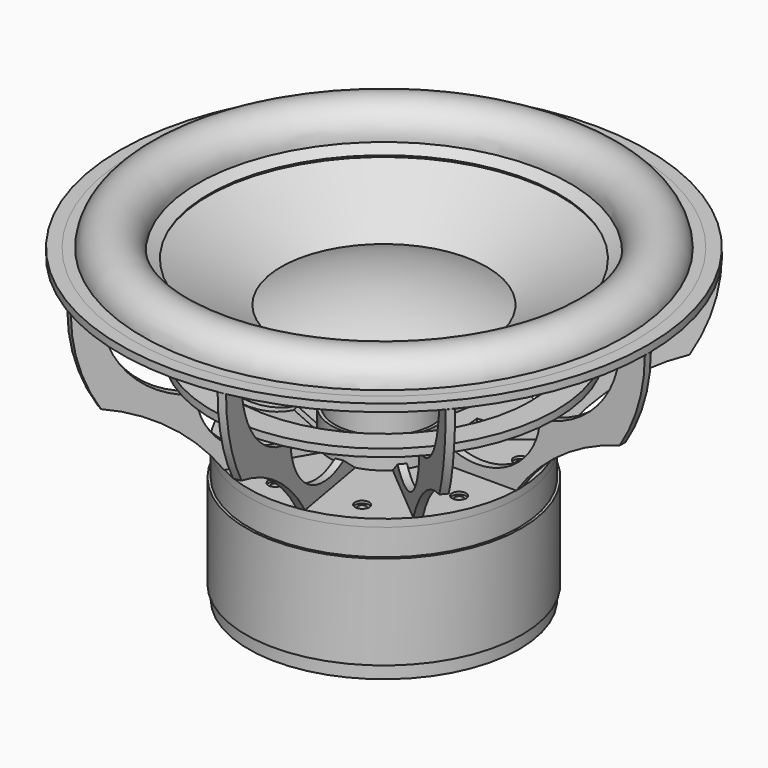
from build123d import *

# Parameters (mm, degrees)
F1_DEPTH       = 3
F1_DEPTH_BACK  = 3
F2_COUNT       = 9
F0_W           = 10
F0_H           = 6
F0_W_2         = 67.2
F0_H_2         = 24.2
F0_W_3         = 2.556
F0_H_3         = 78.232
F0_W_4         = 65.2
F0_H_4         = 21
F6_D           = 6.6
F6_CBORE_D     = 11.25
F6_CBORE_DEPTH = 2


with BuildPart() as f1:
    # F0 (on Front) → F1 (new body, two sides)
    with BuildSketch(Plane.XZ) as f1_sk:
        Polygon((58.0507536311, 12), (42.8, 0), (58.0507536311, 0), align=None)
        with BuildLine():
            Line((58.0507536311, 12), (58.0507536311, 0))
            Line((58.0507536311, 0), (108, 0))
            ThreePointArc((108, 0), (143.9710924133, 36.620389209), (190.461065962, 58.384))
            ThreePointArc((190.461065962, 58.384), (205.4649992375, 91.940728737), (210.5999171392, 128.3385950948))
            Line((210.5999171392, 128.3385950948), (190.5999171392, 128.3385950948))
            ThreePointArc((190.5999171392, 128.3385950948), (175.6594345799, 84.2744472754), (137, 58.384))
            Line((137, 58.384), (127, 58.384))
            ThreePointArc((127, 58.384), (104.8750186644, 16.8344090549), (58.0507536311, 12))
        make_face()
    extrude(amount=F1_DEPTH)
    extrude(f1_sk.sketch, amount=-F1_DEPTH_BACK)


with BuildPart() as f2_1:
    # F2: instance of F1
    add(f1.part.rotate(Axis((0, 0, 16.1796551943), (0, 0, 1)), 1 * 360 / F2_COUNT))


with BuildPart() as f2_2:
    # F2: instance of F1
    add(f1.part.rotate(Axis((0, 0, 16.1796551943), (0, 0, 1)), 2 * 360 / F2_COUNT))


with BuildPart() as f2_3:
    # F2: instance of F1
    add(f1.part.rotate(Axis((0, 0, 16.1796551943), (0, 0, 1)), 3 * 360 / F2_COUNT))


with BuildPart() as f2_4:
    # F2: instance of F1
    add(f1.part.rotate(Axis((0, 0, 16.1796551943), (0, 0, 1)), 4 * 360 / F2_COUNT))


with BuildPart() as f2_5:
    # F2: instance of F1
    add(f1.part.rotate(Axis((0, 0, 16.1796551943), (0, 0, 1)), 5 * 360 / F2_COUNT))


with BuildPart() as f2_6:
    # F2: instance of F1
    add(f1.part.rotate(Axis((0, 0, 16.1796551943), (0, 0, 1)), 6 * 360 / F2_COUNT))


with BuildPart() as f2_7:
    # F2: instance of F1
    add(f1.part.rotate(Axis((0, 0, 16.1796551943), (0, 0, 1)), 7 * 360 / F2_COUNT))


with BuildPart() as f2_8:
    # F2: instance of F1
    add(f1.part.rotate(Axis((0, 0, 16.1796551943), (0, 0, 1)), 8 * 360 / F2_COUNT))


with BuildPart() as f3:
    # F0 (on Front) → F3 (revolve)
    with BuildSketch(Plane.XZ):
        Polygon((58.0507536311, 0), (42.8, 0), (42.8, -6), (108, -6), (108, 0), align=None)
    revolve(axis=Axis((0, 0, 16.1796551943), (0, 0, 1)))

    # F6 (through all)
    with Locations(Plane.XY):
        with Locations((-90, 0), (84.5723358707, -30.7818128993), (45, -77.9422863406), (-15.62833599, -88.6326977711), (-68.9439998807, -57.8508848718), (84.5723358707, 30.7818128993), (-15.62833599, 88.6326977711), (-68.9439998807, 57.8508848718), (45, 77.9422863406)):
            CounterBoreHole(F6_D / 2, F6_CBORE_D / 2, F6_CBORE_DEPTH)


with BuildPart() as f3b:
    # F0 (on Front) → F3, piece 2 (revolve)
    with BuildSketch(Plane.XZ):
        Polygon((150.5999171392, 128.3385950948), (150.5999171392, 130.0313115072), (140.5709525223, 124.7868082016), (82, 94.1579680523), (80.0877188873, 93.1579680523), (39.1, 71.7240279195), (39.1, 70.0313115072), align=None)
    revolve(axis=Axis((0, 0, 16.1796551943), (0, 0, 1)))


with BuildPart() as f3c:
    # F0 (on Front) → F3, piece 3 (revolve)
    with BuildSketch(Plane.XZ):
        Polygon((190.5999171392, 128.3385950948), (210.5999171392, 128.3385950948), (210.5999171392, 134.3385950948), (200.5999171392, 134.3385950948), (200.5999171392, 132.3385950948), (190.5999171392, 132.3385950948), align=None)
    revolve(axis=Axis((0, 0, 16.1796551943), (0, 0, 1)))


with BuildPart() as f3d:
    # F0 (on Front) → F3, piece 4 (revolve)
    with BuildSketch(Plane.XZ):
        with Locations((132, 61.384)):
            Rectangle(F0_W, F0_H)
        with Locations((122, 61.384)):
            Rectangle(F0_W, F0_H)
    revolve(axis=Axis((0, 0, 16.1796551943), (0, 0, 1)))


with BuildPart() as f3e:
    # F0 (on Front) → F3, piece 5 (revolve)
    with BuildSketch(Plane.XZ):
        Polygon((108, -27), (42.8, -27), (42.8, -52.4), (110, -52.4), (110, -27), align=None)
        with Locations((76.4, -64.5)):
            Rectangle(F0_W_2, F0_H_2)
        Polygon((110, -76.6), (42.8, -76.6), (42.8, -102), (108, -102), (110, -102), align=None)
    revolve(axis=Axis((0, 0, 16.1796551943), (0, 0, 1)))


with BuildPart() as f3f:
    # F0 (on Front) → F3, piece 6 (revolve)
    with BuildSketch(Plane.XZ):
        with Locations((40.378, -16.5)):
            Rectangle(F0_W_3, F0_H_3)
    revolve(axis=Axis((0, 0, 16.1796551943), (0, 0, 1)))


with BuildPart() as f4:
    # F0 (on Front) → F4 (revolve)
    with BuildSketch(Plane.XZ):
        Polygon((39.1, 22.616), (39.1, 70.0313115072), (39.1, 71.7240279195), (38.1, 71.7240279195), (38.1, -55.616), (39.1, -55.616), align=None)
    revolve(axis=Axis((0, 0, 16.1796551943), (0, 0, 1)))


with BuildPart() as f4b:
    # F0 (on Front) → F4, piece 2 (revolve)
    with BuildSketch(Plane.XZ):
        with BuildLine():
            Line((80.0877188873, 93.1579680523), (82, 94.1579680523))
            ThreePointArc((82, 94.1579680523), (42.0377764011, 108.0245049603), (0, 112.7240279195))
            Line((0, 112.7240279195), (0, 111.7240279195))
            ThreePointArc((0, 111.7240279195), (41.0580654121, 106.8159403849), (80.0877188873, 93.1579680523))
        make_face()
    revolve(axis=Axis((0, 0, 16.1796551943), (0, 0, 1)))


with BuildPart() as f4c:
    # F0 (on Front) → F4, piece 3 (revolve)
    with BuildSketch(Plane.XZ):
        with Locations((75.4, -16.5)):
            Rectangle(F0_W_4, F0_H_4)
    revolve(axis=Axis((0, 0, 16.1796551943), (0, 0, 1)))


with BuildPart() as f4d:
    # F0 (on Front) → F4, piece 4 (revolve)
    with BuildSketch(Plane.XZ):
        Polygon((108, -102), (42.8, -102), (37.5, -102), (20, -102), (20, -123), (83.0537039877, -123), (108, -112.7044326116), align=None)
        with BuildLine():
            Line((20, -102), (37.5, -102))
            Line((37.5, -102), (37.5, 3.3759615954))
            Line((37.5, 3.3759615954), (35.5, 3.3759615954))
            ThreePointArc((35.5, 3.3759615954), (29.0575749491, -3.4736547322), (20, -6))
            Line((20, -6), (20, -102))
        make_face()
    revolve(axis=Axis((0, 0, 16.1796551943), (0, 0, 1)))


with BuildPart() as f4e:
    # F0 (on Front) → F4, piece 5 (revolve)
    with BuildSketch(Plane.XZ):
        with BuildLine():
            ThreePointArc((150.5999171392, 130.0313115072), (169.3778132577, 152.3718396994), (190.5999171392, 132.3385950948))
            Line((190.5999171392, 132.3385950948), (200.5999171392, 132.3385950948))
            Line((200.5999171392, 132.3385950948), (200.5999171392, 134.3385950948))
            Line((200.5999171392, 134.3385950948), (196.5499585696, 134.3385950948))
            Line((196.5499585696, 134.3385950948), (192.5, 134.3385950948))
            ThreePointArc((192.5, 134.3385950948), (168.9603284106, 154.3399188737), (148.5056502069, 131.1930998476))
            Line((148.5056502069, 131.1930998476), (139.6441540398, 126.559107435))
            Line((139.6441540398, 126.559107435), (140.5709525223, 124.7868082016))
            Line((140.5709525223, 124.7868082016), (150.5999171392, 130.0313115072))
        make_face()
    revolve(axis=Axis((0, 0, 16.1796551943), (0, 0, 1)))


solid = Compound([f1.part, f2_1.part, f2_2.part, f2_3.part, f2_4.part, f2_5.part, f2_6.part, f2_7.part, f2_8.part, f3.part, f3b.part, f3c.part, f3d.part, f3e.part, f3f.part, f4.part, f4b.part, f4c.part, f4d.part, f4e.part])
